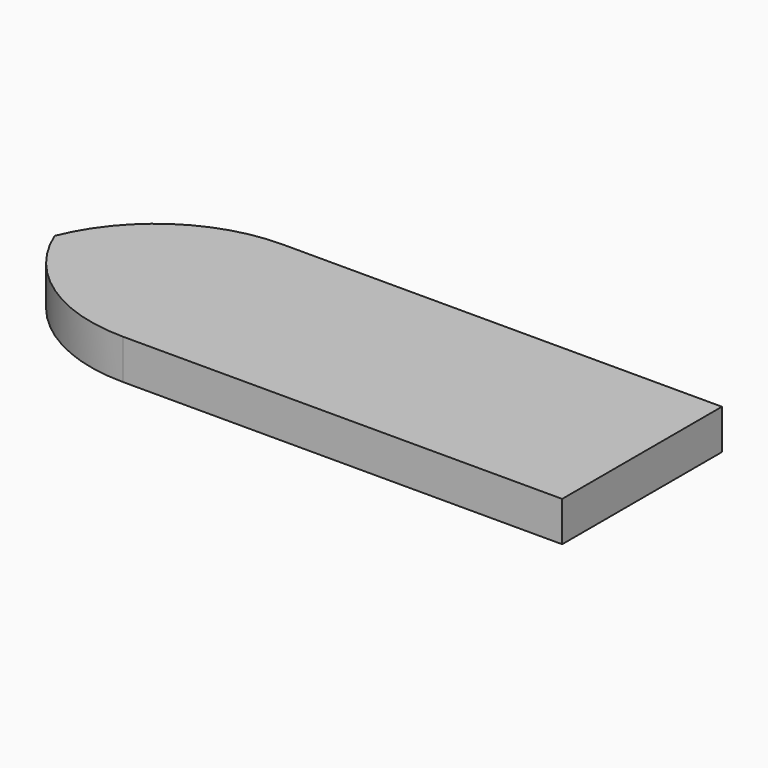
from build123d import *

# Parameters (mm, degrees)
F0_W        = 75
F0_H        = 25
F1_DEPTH    = 5
F2_T1_DEPTH = 105


# Not quite as in the source:
# - a fillet or chamfer that OpenCascade refuses, or shapes differently, is made with other operations: its cross-section is extruded or revolved along the edge and cut away or added


with BuildPart() as f1:
    # F0 (on Top) → F1 (new body)
    with BuildSketch(Plane.XY):
        Rectangle(F0_W, F0_H)
    extrude(amount=F1_DEPTH)

    # F2: fillet of radius 20 on 2 edges, made by hand

    # F2_s2 → F2_t1 (cut)
    with BuildSketch(Plane.XY.offset(-50)):
        with BuildLine():
            ThreePointArc((-17.5, 12.5), (-31.6421356237, 6.6421356237), (-37.5, -7.5))
            Line((-37.5, -7.5), (-37.5, 12.5))
            Line((-37.5, 12.5), (-17.5, 12.5))
        make_face()
        with BuildLine():
            ThreePointArc((-37.5, 7.5), (-31.6421356237, -6.6421356237), (-17.5, -12.5))
            Line((-17.5, -12.5), (-37.5, -12.5))
            Line((-37.5, -12.5), (-37.5, 7.5))
        make_face()
    extrude(amount=F2_T1_DEPTH, mode=Mode.SUBTRACT)


solid = f1.part
